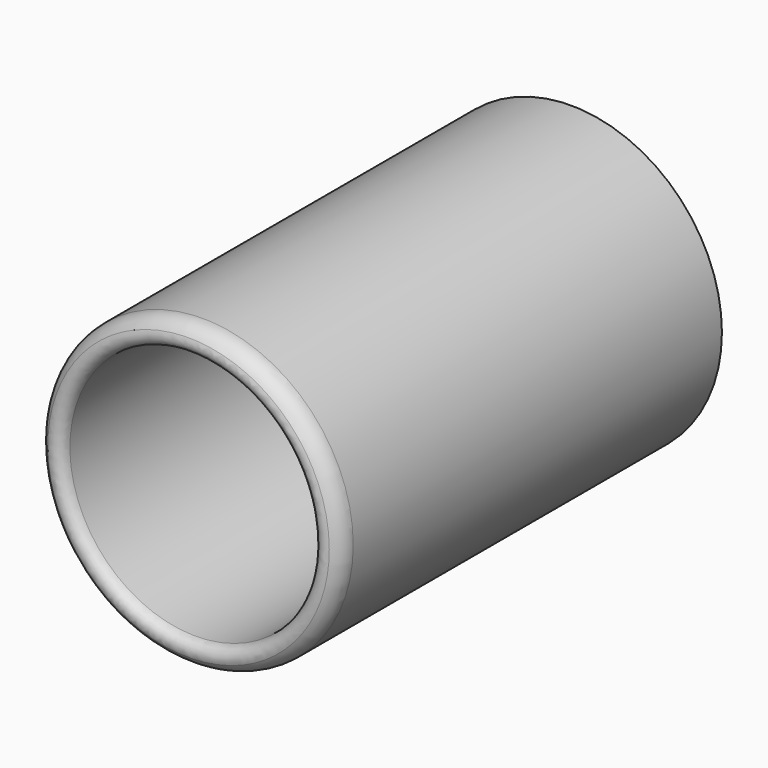
from build123d import *

# Parameters (mm, degrees)
F0_R     = 38.1
F0_R_2   = 31.75
F1_DEPTH = 121.539
F2_DEPTH = 9.525
F3_R     = 5.08
F4_R     = 2.54


# Not quite as in the source:
# - a length typed as a fraction of an inch, garbled in the dataset ("3 / 203.2 mm" for 3/8 in), is restored


with BuildPart() as f1:
    # F0 (on Front) → F1 (new body)
    with BuildSketch(Plane.XZ):
        Circle(F0_R)
        Circle(F0_R_2, mode=Mode.SUBTRACT)
    extrude(amount=F1_DEPTH)

    # F0 (on Front) → F2 (join)
    with BuildSketch(Plane.XZ):
        Circle(F0_R_2)
    extrude(amount=F2_DEPTH)

    # F3
    f3_edges = [f1.edges().sort_by_distance(p)[0] for p in [
        (-38.1, -121.539, 0),
    ]]
    fillet(f3_edges, radius=F3_R)

    # F4
    f4_edges = [f1.edges().sort_by_distance(p)[0] for p in [
        (-31.75, -121.539, 0),
    ]]
    fillet(f4_edges, radius=F4_R)


solid = f1.part
